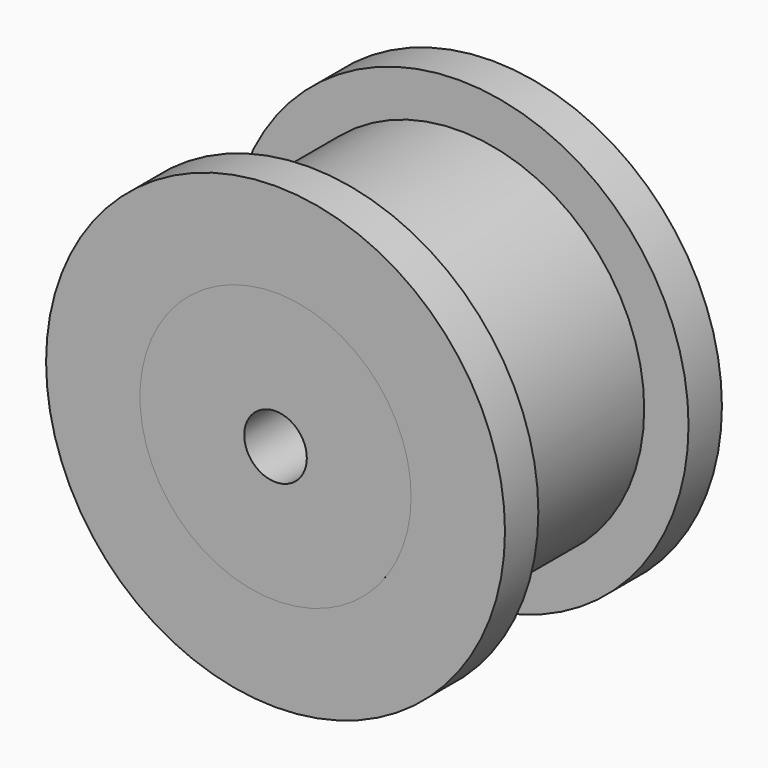
from build123d import *

# Parameters (mm, degrees)
F0_R      = 11
F0_R_2    = 2.5
F1_DEPTH  = 2
F2_R      = 8.875
F2_R_2    = 2.5
F3_DEPTH  = 9
F4_R      = 11
F4_R_2    = 8.875
F4_R_3    = 2.5
F5_DEPTH  = 2
F6_R      = 6.5
F6_R_2    = 1.5
F7_DEPTH  = 2
F8_R      = 4.5
F8_R_2    = 1.5
F9_DEPTH  = 9
F10_R     = 6.5
F10_R_2   = 4.5
F10_R_3   = 1.5
F11_DEPTH = 2


with BuildPart() as f1:
    # F0 (on Front) → F1 (new body)
    with BuildSketch(Plane.XZ):
        Circle(F0_R)
        Circle(F0_R_2, mode=Mode.SUBTRACT)
    extrude(amount=F1_DEPTH)

    # F2 (on face) → F3 (join)
    with BuildSketch(Plane.XZ.offset(2)):
        Circle(F2_R)
        Circle(F2_R_2, mode=Mode.SUBTRACT)
    extrude(amount=F3_DEPTH)

    # F4 (on face) → F5 (join)
    with BuildSketch(Plane.XZ.offset(11)):
        Circle(F4_R)
        Circle(F4_R_2, mode=Mode.SUBTRACT)
        Circle(F4_R_2)
        Circle(F4_R_3, mode=Mode.SUBTRACT)
    extrude(amount=F5_DEPTH)


with BuildPart() as f7:
    # F6 (on Front) → F7 (new body)
    with BuildSketch(Plane.XZ):
        Circle(F6_R)
        Circle(F6_R_2, mode=Mode.SUBTRACT)
    extrude(amount=F7_DEPTH)

    # F8 (on face) → F9 (join)
    with BuildSketch(Plane.XZ.offset(2)):
        Circle(F8_R)
        Circle(F8_R_2, mode=Mode.SUBTRACT)
    extrude(amount=F9_DEPTH)

    # F10 (on face) → F11 (join)
    with BuildSketch(Plane.XZ.offset(11)):
        Circle(F10_R)
        Circle(F10_R_2, mode=Mode.SUBTRACT)
        Circle(F10_R_2)
        Circle(F10_R_3, mode=Mode.SUBTRACT)
    extrude(amount=F11_DEPTH)


solid = Compound([f1.part, f7.part])
